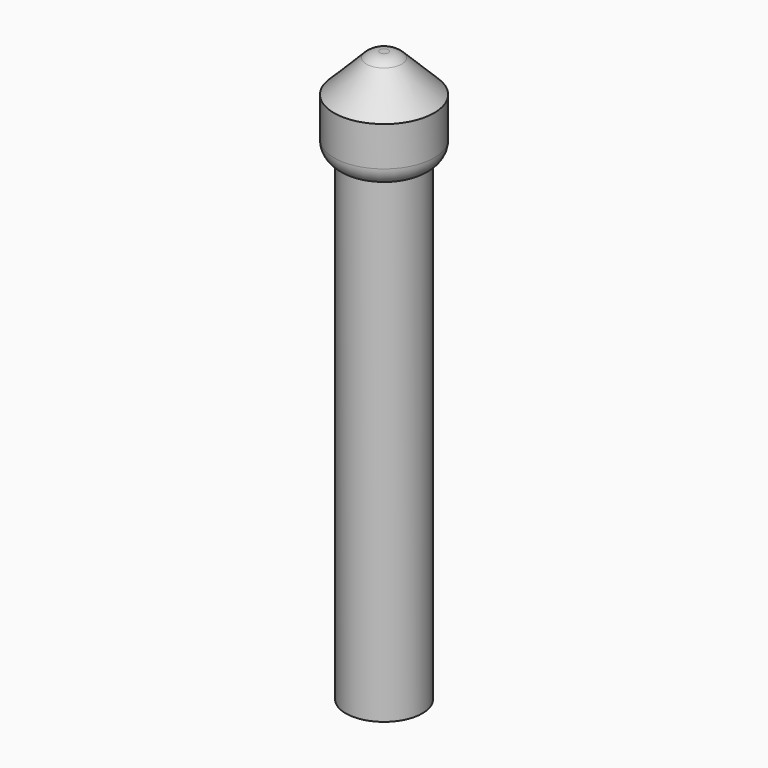
from build123d import *

# Parameters (mm, degrees)
F4_R     = 10.2299469816
F0_DEPTH = 127
F1_R     = 13.3830980952
F5_DEPTH = 25.4
F3_SIZE  = 10.16
F6_R     = 5.08


# Not quite as in the source:
# - a fillet or chamfer that OpenCascade refuses, or shapes differently, is made with other operations: its cross-section is extruded or revolved along the edge and cut away or added


with BuildPart() as f0:
    # F4 (on Top) → F0 (new body)
    with BuildSketch(Plane.XY):
        Circle(F4_R)
    extrude(amount=F0_DEPTH)

    # F1 (on face) → F5 (join)
    with BuildSketch(Plane.XY.offset(127)):
        Circle(F1_R)
    extrude(amount=F5_DEPTH)

    # F2: fillet of radius 5.08 on 1 edges, made by hand

    # F2_s1 → F2_t2 (revolve, cut)
    with BuildSketch(Plane.XZ):
        with BuildLine():
            ThreePointArc((13.3830980952, 131.7003886402), (12.5217941226, 128.870370296), (10.2299469816, 127))
            Line((10.2299469816, 127), (13.3830980952, 127))
            Line((13.3830980952, 127), (13.3830980952, 131.7003886402))
        make_face()
    revolve(axis=Axis((0, 0, 127), (0, 0, 1)), mode=Mode.SUBTRACT)

    # F3
    f3_edges = [f0.edges().sort_by_distance(p)[0] for p in [
        (-13.383098, 0, 152.4),
    ]]
    chamfer(f3_edges, length=F3_SIZE)

    # F6
    f6_edges = [f0.edges().sort_by_distance(p)[0] for p in [
        (-3.223098, 0, 152.4),
    ]]
    fillet(f6_edges, radius=F6_R)


solid = f0.part
